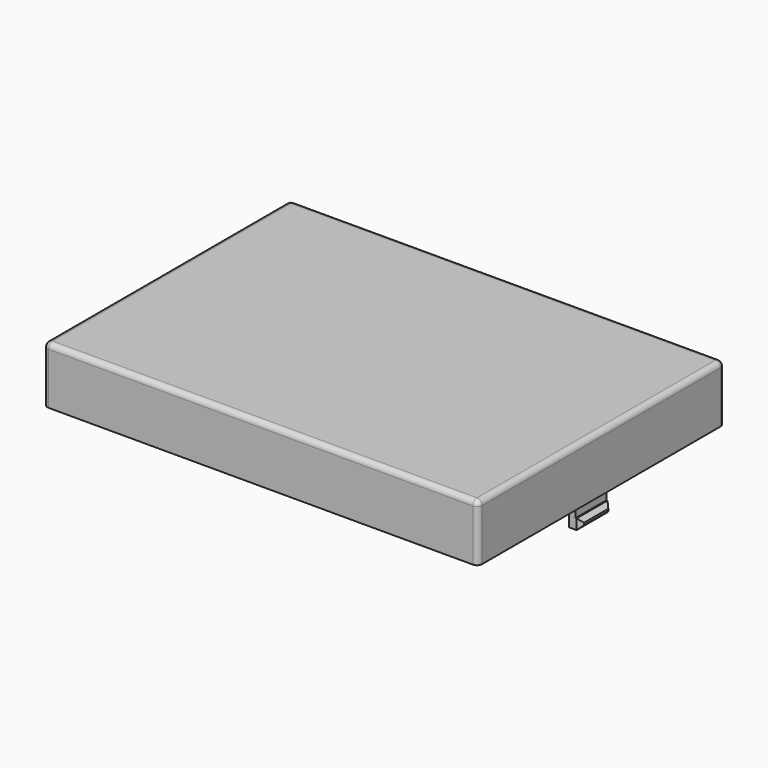
from build123d import *

# Parameters (mm, degrees)
F0_W      = 84.25
F0_H      = 59.75
F1_DEPTH  = 11
F2_W      = 80.25
F2_H      = 55.75
F3_DEPTH  = 9
F4_W      = 82.25
F4_H      = 57.75
F4_W_2    = 80.25
F4_H_2    = 55.75
F5_DEPTH  = 2
F6_W      = 7.5
F6_H      = 7
F7_DEPTH  = 1.25
F8_R      = 1
F9_W      = 7.5
F9_H      = 2
F10_DEPTH = 1
F11_SIZE  = 0.8


with BuildPart() as f1:
    # F0 (on Top) → F1 (new body)
    with BuildSketch(Plane.XY):
        Rectangle(F0_W, F0_H)
    extrude(amount=F1_DEPTH)

    # F2 (on face) → F3 (cut)
    with BuildSketch(Plane(origin=(0, 0, 0), x_dir=(1, 0, 0), z_dir=(0, 0, -1))):
        Rectangle(F2_W, F2_H)
    extrude(amount=-F3_DEPTH, mode=Mode.SUBTRACT)

    # F4 (on face) → F5 (cut)
    with BuildSketch(Plane(origin=(0, 0, 0), x_dir=(1, 0, 0), z_dir=(0, 0, -1))):
        Rectangle(F4_W, F4_H)
        Rectangle(F4_W_2, F4_H_2, mode=Mode.SUBTRACT)
    extrude(amount=-F5_DEPTH, mode=Mode.SUBTRACT)

    # F6 (on face) → F7 (join)
    with BuildSketch(Plane.YZ.offset(-40.125)):
        with Locations((0, -1.5)):
            Rectangle(F6_W, F6_H)
        with Locations((0, 5.5)):
            Rectangle(F6_W, F6_H)
    extrude(amount=F7_DEPTH)

    # F8
    f8_edges = [f1.edges().sort_by_distance(p)[0] for p in [
        (-42.125, -29.875, 5.5),
        (42.125, -29.875, 5.5),
        (-42.125, 29.875, 5.5),
        (42.125, 29.875, 5.5),
        (0, 29.875, 11),
        (-42.125, 0, 11),
        (0, -29.875, 11),
        (42.125, 0, 11),
    ]]
    fillet(f8_edges, radius=F8_R)

    # F9 (on face) → F10 (join)
    with BuildSketch(Plane(origin=(-40.125, 0, 0), x_dir=(0, -1, 0), z_dir=(-1, 0, 0))):
        with Locations((0, -4)):
            Rectangle(F9_W, F9_H)
    extrude(amount=F10_DEPTH)

    # F11
    f11_edges = [f1.edges().sort_by_distance(p)[0] for p in [
        (-41.125, 0, -3),
        (-41.125, 3.75, -4),
        (-41.125, 0, -5),
        (-41.125, -3.75, -4),
    ]]
    chamfer(f11_edges, length=F11_SIZE)

    # F12: F1 across plane


with BuildPart() as f1_1:
    add(f1.part)
    add(f1.part.mirror(Plane.YZ))


solid = f1_1.part
